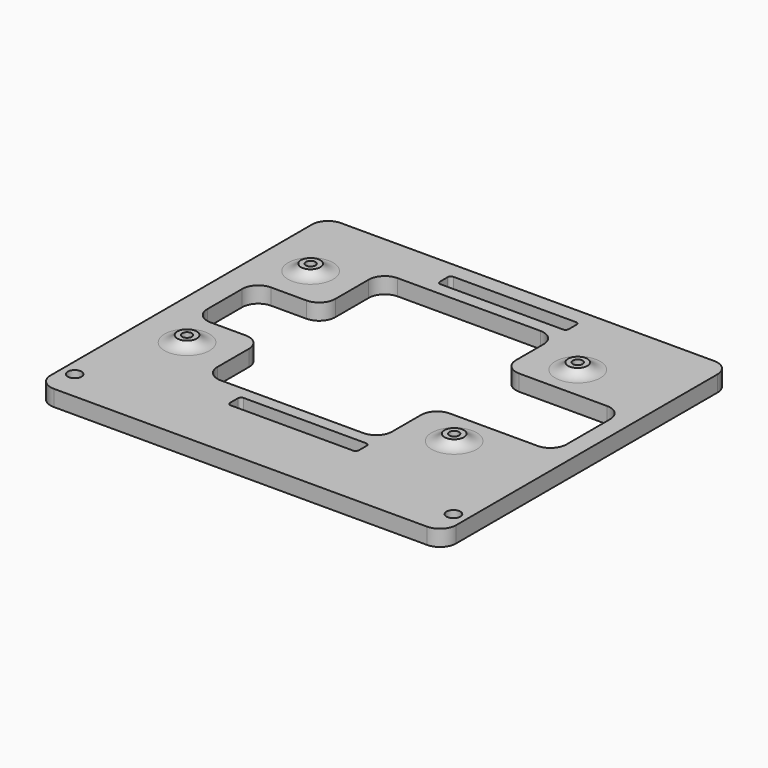
from build123d import *

# Parameters (mm, degrees)
F0_R     = 2.15
F0_R_2   = 3
F0_R_3   = 1.5
F0_R_4   = 5
F1_DEPTH = 5
F2_R     = 1
F3_R     = 5
F4_DEPTH = 7
F6_W     = 20.916191861
F6_H     = 23.5347189009
F6_W_2   = 37.2305270284
F6_H_2   = 26.8968194723
F7_DEPTH = 25
F8_R     = 5


# Not quite as in the source:
# - a fillet or chamfer that OpenCascade refuses, or shapes differently, is made with other operations: its cross-section is extruded or revolved along the edge and cut away or added


with BuildPart() as f1:
    # F0 (on Top) → F1 (new body)
    with BuildSketch(Plane.XY):
        Polygon((-49.7560231508, 20), (-49.7560231508, 0), (76.2439768492, 0), (76.2439768492, 20), (33.2439768492, 20), (-6.7560231508, 20), align=None)
        with Locations((-45.6060231508, 9.15)):
            Circle(F0_R, mode=Mode.SUBTRACT)
        with Locations((72.0939768492, 9.15)):
            Circle(F0_R, mode=Mode.SUBTRACT)
        Polygon((-49.7560231508, 106.5), (-49.7560231508, 20), (-6.7560231508, 20), (-6.7560231508, 25), (33.2439768492, 25), (33.2439768492, 20), (76.2439768492, 20), (76.2439768492, 106.5), (33.2439768492, 106.5), (33.2439768492, 101.5), (-6.7560231508, 101.5), (-6.7560231508, 106.5), align=None)
        with Locations((-34.7560231508, 39.25)):
            Circle(F0_R_2, mode=Mode.SUBTRACT)
        with Locations((3.2439768492, 53.25)):
            Circle(F0_R_3, mode=Mode.SUBTRACT)
        with Locations((23.2439768492, 53.25)):
            Circle(F0_R_3, mode=Mode.SUBTRACT)
        with Locations((48.2439768492, 39.25)):
            Circle(F0_R_2, mode=Mode.SUBTRACT)
        with Locations((3.2439768492, 73.25)):
            Circle(F0_R_3, mode=Mode.SUBTRACT)
        with Locations((-34.7560231508, 87.25)):
            Circle(F0_R_2, mode=Mode.SUBTRACT)
        with Locations((13.2439768492, 63.25)):
            Circle(F0_R_4, mode=Mode.SUBTRACT)
        with Locations((23.2439768492, 73.25)):
            Circle(F0_R_3, mode=Mode.SUBTRACT)
        with Locations((48.2439768492, 87.25)):
            Circle(F0_R_2, mode=Mode.SUBTRACT)
        Polygon((-49.7560231508, 111.5), (-49.7560231508, 106.5), (-6.7560231508, 106.5), (33.2439768492, 106.5), (76.2439768492, 106.5), (76.2439768492, 111.5), align=None)
        with Locations((-34.7560231508, 39.25)):
            Circle(F0_R_2)
        with Locations((-34.7560231508, 39.25)):
            Circle(F0_R_3, mode=Mode.SUBTRACT)
        with Locations((-34.7560231508, 87.25)):
            Circle(F0_R_2)
        with Locations((-34.7560231508, 87.25)):
            Circle(F0_R_3, mode=Mode.SUBTRACT)
        with Locations((48.2439768492, 39.25)):
            Circle(F0_R_2)
        with Locations((48.2439768492, 39.25)):
            Circle(F0_R_3, mode=Mode.SUBTRACT)
        with Locations((48.2439768492, 87.25)):
            Circle(F0_R_2)
        with Locations((48.2439768492, 87.25)):
            Circle(F0_R_3, mode=Mode.SUBTRACT)
        with Locations((13.2439768492, 63.25)):
            Circle(F0_R_4)
        with Locations((3.2439768492, 73.25)):
            Circle(F0_R_3)
        with Locations((3.2439768492, 53.25)):
            Circle(F0_R_3)
        with Locations((23.2439768492, 53.25)):
            Circle(F0_R_3)
        with Locations((23.2439768492, 73.25)):
            Circle(F0_R_3)
    extrude(amount=F1_DEPTH)

    # F2
    f2_edges = [f1.edges().sort_by_distance(p)[0] for p in [
        (-6.756023, 25, 2.5),
        (33.243977, 25, 2.5),
        (-6.756023, 20, 2.5),
        (33.243977, 20, 2.5),
        (-6.756023, 101.5, 2.5),
        (-6.756023, 106.5, 2.5),
        (33.243977, 106.5, 2.5),
        (33.243977, 101.5, 2.5),
    ]]
    fillet(f2_edges, radius=F2_R)

    # F3
    f3_edges = [f1.edges().sort_by_distance(p)[0] for p in [
        (-49.756023, 0, 2.5),
        (76.243977, 0, 2.5),
        (76.243977, 111.5, 2.5),
        (-49.756023, 111.5, 2.5),
    ]]
    fillet(f3_edges, radius=F3_R)

    # F0 (on Top) → F4 (join)
    with BuildSketch(Plane.XY):
        with Locations((-34.7560231508, 87.25)):
            Circle(F0_R_2)
        with Locations((-34.7560231508, 87.25)):
            Circle(F0_R_3, mode=Mode.SUBTRACT)
        with Locations((-34.7560231508, 39.25)):
            Circle(F0_R_2)
        with Locations((-34.7560231508, 39.25)):
            Circle(F0_R_3, mode=Mode.SUBTRACT)
        with Locations((48.2439768492, 87.25)):
            Circle(F0_R_2)
        with Locations((48.2439768492, 87.25)):
            Circle(F0_R_3, mode=Mode.SUBTRACT)
        with Locations((48.2439768492, 39.25)):
            Circle(F0_R_2)
        with Locations((48.2439768492, 39.25)):
            Circle(F0_R_3, mode=Mode.SUBTRACT)
    extrude(amount=F4_DEPTH)

    # F5: fillet of radius 5 on 4 edges, made by hand

    # F5_s1 → F5_t2 (revolve)
    with BuildSketch(Plane.XZ.offset(-87.25)):
        with BuildLine():
            ThreePointArc((-27.7560231508, 5), (-29.9920911283, 5.527864045), (-31.7560231508, 7))
            Line((-31.7560231508, 7), (-31.7560231508, 5))
            Line((-31.7560231508, 5), (-27.7560231508, 5))
        make_face()
    revolve(axis=Axis((-34.7560231508, 87.25, 5), (0, 0, -1)))

    # F5_s3 → F5_t4 (revolve)
    with BuildSketch(Plane.XZ.offset(-39.25)):
        with BuildLine():
            ThreePointArc((-27.7560231508, 5), (-29.9920911283, 5.527864045), (-31.7560231508, 7))
            Line((-31.7560231508, 7), (-31.7560231508, 5))
            Line((-31.7560231508, 5), (-27.7560231508, 5))
        make_face()
    revolve(axis=Axis((-34.7560231508, 39.25, 5), (0, 0, -1)))

    # F5_s5 → F5_t6 (revolve)
    with BuildSketch(Plane.XZ.offset(-39.25)):
        with BuildLine():
            ThreePointArc((55.2439768492, 5), (53.0079088717, 5.527864045), (51.2439768492, 7))
            Line((51.2439768492, 7), (51.2439768492, 5))
            Line((51.2439768492, 5), (55.2439768492, 5))
        make_face()
    revolve(axis=Axis((48.2439768492, 39.25, 5), (0, 0, -1)))

    # F5_s7 → F5_t8 (revolve)
    with BuildSketch(Plane.XZ.offset(-87.25)):
        with BuildLine():
            ThreePointArc((51.2439768492, 7), (53.0079088717, 5.527864045), (55.2439768492, 5))
            Line((55.2439768492, 5), (51.2439768492, 5))
            Line((51.2439768492, 5), (51.2439768492, 7))
        make_face()
    revolve(axis=Axis((48.2439768492, 87.25, 5), (0, 0, -1)))

    # F6 (on face) → F7 (cut)
    with BuildSketch(Plane.XY.offset(5)):
        Polygon((33.4173643496, 97.5044071674), (-20.9036788438, 97.5044071674), (-20.9036788438, 74.5087079704), (-20.9036788438, 50.9739890695), (-20.9036788438, 28.7407264113), (33.4173643496, 28.7407264113), (33.4173643496, 49.8894378543), (33.4173643496, 76.7862573266), align=None)
        with Locations((-31.3617747743, 62.7413485199)):
            Rectangle(F6_W, F6_H)
        with Locations((52.0326278638, 63.3378475904)):
            Rectangle(F6_W_2, F6_H_2)
    extrude(amount=-F7_DEPTH, mode=Mode.SUBTRACT)

    # F8
    f8_edges = [f1.edges().sort_by_distance(p)[0] for p in [
        (-20.903679, 74.508708, 2.5),
        (33.417364, 76.786257, 2.5),
        (33.417364, 49.889438, 2.5),
        (-20.903679, 50.973989, 2.5),
        (-41.819871, 50.973989, 2.5),
        (-41.819871, 74.508708, 2.5),
        (-20.903679, 97.504407, 2.5),
        (33.417364, 97.504407, 2.5),
        (70.647891, 76.786257, 2.5),
        (70.647891, 49.889438, 2.5),
        (33.417364, 28.740726, 2.5),
        (-20.903679, 28.740726, 2.5),
    ]]
    fillet(f8_edges, radius=F8_R)


solid = f1.part
